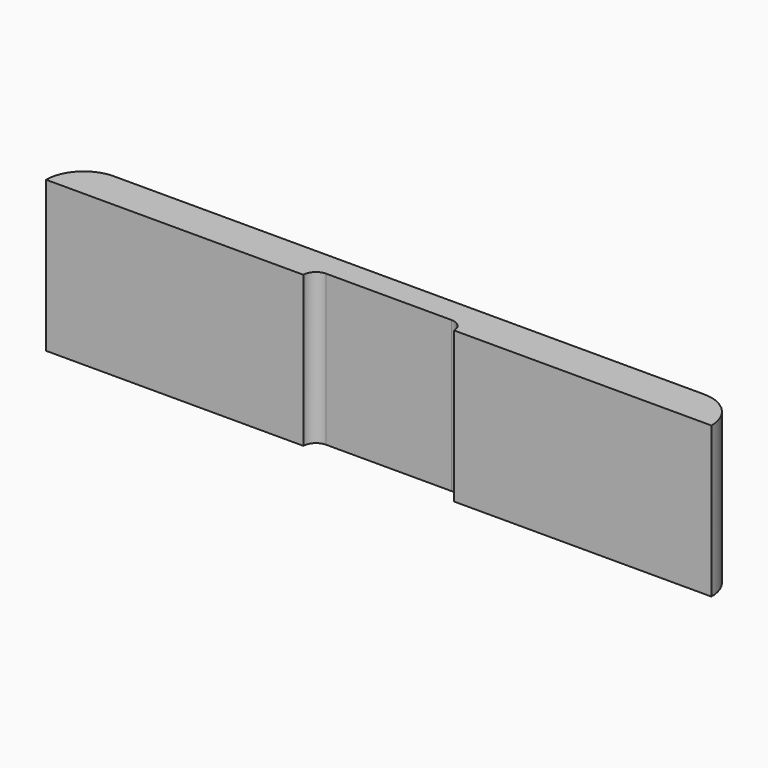
from build123d import *

# Parameters (mm, degrees)
F1_DEPTH = 12
F2_R     = 0.99999
F3_R     = 2.99999


# Not quite as in the source:
# - a fillet or chamfer is up to 0.001 mm smaller than in the source, because OpenCascade refuses the exact size


with BuildPart() as f1:
    # F0 (on Top) → F1 (new body)
    with BuildSketch(Plane.XY):
        Polygon((23.3803613689, 1.1605409955), (5.8803613689, 1.1605409955), (5.8803613689, -1.8394590045), (26.3803613689, -1.8394590045), (26.3803613689, -0.8394590045), (38.3803613689, -0.8394590045), (38.3803613689, -1.8394590045), (58.8803613689, -1.8394590045), (58.8803613689, 1.1605409955), (41.3803613689, 1.1605409955), align=None)
    extrude(amount=F1_DEPTH)

    # F2 (radius 1 in the source; OpenCascade refuses exactly that, so slightly less here)
    f2_edges = [f1.edges().sort_by_distance(p)[0] for p in [
        (38.380361, -0.839459, 6),
        (26.380361, -0.839459, 6),
    ]]
    fillet(f2_edges, radius=F2_R)

    # F3 (radius 3 in the source; OpenCascade refuses exactly that, so slightly less here)
    f3_edges = [f1.edges().sort_by_distance(p)[0] for p in [
        (5.880361, 1.160541, 6),
        (58.880361, 1.160541, 6),
    ]]
    fillet(f3_edges, radius=F3_R)


solid = f1.part
